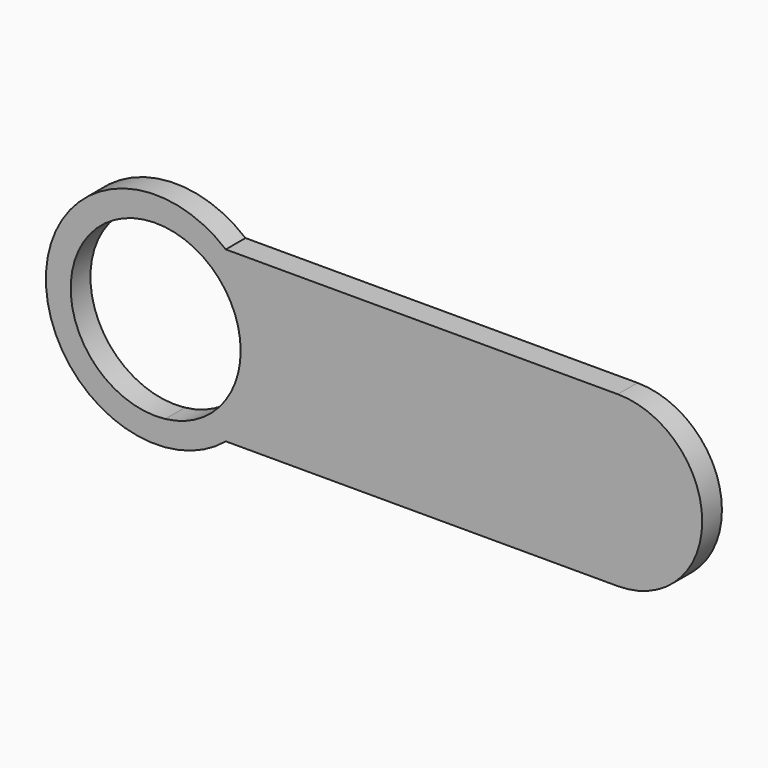
from build123d import *

# Parameters (mm, degrees)
F1_DEPTH = 5


# Not quite as in the source:
# - the program builds the solid bodies; features that only make, move or delete a surface that nothing else refers to are left out


with BuildPart() as f1:
    # F0 (on Front) → F1 (new body)
    with BuildSketch(Plane.XZ):
        with BuildLine():
            ThreePointArc((-38.5628677204, -8.4046955637), (-42.950748766, -19.8978357544), (-53.8815692168, -25.542562124))
            Line((-53.8815692168, -25.542562124), (-41.5648788357, -25.542562124))
            ThreePointArc((-41.5648788357, -25.542562124), (-35.6343803196, -17.869848935), (-33.5243537826, -8.4046955637))
            ThreePointArc((-33.5243537826, -8.4046955637), (-35.6391308825, 1.0705767284), (-41.5820798093, 8.7474527367))
            Line((-41.5820798093, 8.7474527367), (-54.0131150031, 8.7474527367))
            ThreePointArc((-54.0131150031, 8.7474527367), (-42.9949338553, 3.137686474), (-38.5628677204, -8.4046955637))
        make_face()
        with BuildLine():
            Line((-41.5648788357, -25.542562124), (-53.8815692168, -25.542562124))
            ThreePointArc((-53.8815692168, -25.542562124), (-73.0545080153, -8.4708549583), (-54.0131150031, 8.7474527367))
            Line((-54.0131150031, 8.7474527367), (-41.5820798093, 8.7474527367))
            ThreePointArc((-41.5820798093, 8.7474527367), (-78.0931460515, -8.4158741323), (-41.5648788357, -25.542562124))
        make_face()
        with BuildLine():
            ThreePointArc((-33.5243537826, -8.4046955637), (-35.6343803196, -17.869848935), (-41.5648788357, -25.542562124))
            Line((-41.5648788357, -25.542562124), (37.9639441457, -25.542562124))
            ThreePointArc((37.9639441457, -25.542562124), (55.1089515761, -8.3975546937), (37.9639441457, 8.7474527367))
            Line((37.9639441457, 8.7474527367), (-41.5820798093, 8.7474527367))
            ThreePointArc((-41.5820798093, 8.7474527367), (-35.6391308825, 1.0705767284), (-33.5243537826, -8.4046955637))
        make_face()
        with BuildLine():
            Line((37.9639441457, -20.3371653928), (37.9639441457, -17.8371653928))
            ThreePointArc((37.9639441457, -17.8371653928), (44.7629027111, -8.9185826964), (37.9639441457, 0))
            Line((37.9639441457, 0), (37.9639441457, 2.5))
            ThreePointArc((37.9639441457, 2.5), (48.2332452633, -8.9185826964), (37.9639441457, -20.3371653928))
        make_face(mode=Mode.SUBTRACT)
        with BuildLine():
            ThreePointArc((37.9639441457, 0), (44.7629027111, -8.9185826964), (37.9639441457, -17.8371653928))
            Line((37.9639441457, -17.8371653928), (37.9639441457, -20.3371653928))
            ThreePointArc((37.9639441457, -20.3371653928), (48.2332452633, -8.9185826964), (37.9639441457, 2.5))
            Line((37.9639441457, 2.5), (37.9639441457, 0))
        make_face()
    extrude(amount=F1_DEPTH)


solid = f1.part
